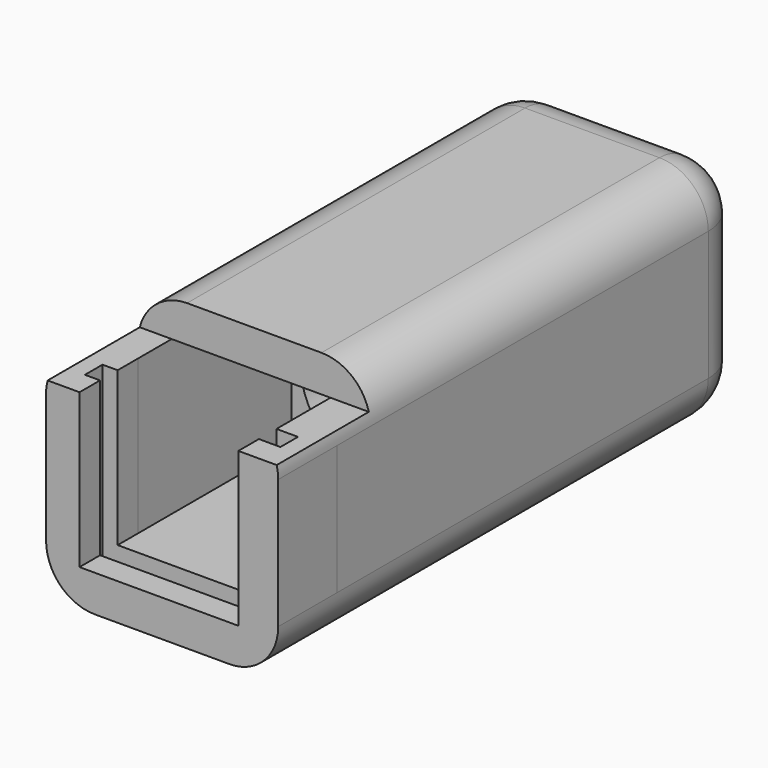
from build123d import *

# Parameters (mm, degrees)
F0_W         = 1.3692331631
F0_H         = 7.834737435
F0_W_2       = 6.5
F0_H_2       = 0.9
F0_W_3       = 0.6192331631
F0_H_3       = 1.05
F0_H_4       = 13.165262565
F0_W_4       = 0.8807668369
F0_W_5       = 1.6307668369
F1_DEPTH     = 0.9
F2_DEPTH     = 1.5
F3_DEPTH     = 7.8
F5_W         = 9.5
F5_H         = 19.2867757659
F6_DEPTH     = 1.5
F7_R         = 3
F8_DEPTH     = 20
F9_T1_DEPTH  = 5.3
F9_T3_DEPTH  = 5.5
F9_T5_DEPTH  = 22.2867757659
F9_T7_DEPTH  = 27
F9_S11_W     = 2
F9_S11_H     = 2
F9_T12_DEPTH = 2
F9_S17_W     = 2
F9_S17_H     = 2
F9_T18_DEPTH = 2
F9_S23_W     = 2
F9_S23_H     = 2
F9_T24_DEPTH = 2
F9_S29_W     = 2
F9_S29_H     = 2
F9_T30_DEPTH = 2
F10_R        = 2.7204865104
F11_DEPTH    = 6


# Not quite as in the source:
# - a fillet or chamfer that OpenCascade refuses, or shapes differently, is made with other operations: its cross-section is extruded or revolved along the edge and cut away or added
# - a feature names something its author has since deleted; it is built from what else it names


with BuildPart() as f1:
    # F0 (on Top) → F1 (new body)
    with BuildSketch(Plane.XY):
        Polygon((-4.75, 1.5), (-4.75, -1.5), (-3.3807668369, -1.5), (-3.3807668369, -0.45), (-4, -0.45), (-4, 0.45), (-3.3807668369, 0.45), (-3.3807668369, 1.5), align=None)
        Polygon((-3.3807668369, -0.45), (-3.3807668369, -1.5), (-3.1192331631, -1.5), (3.1192331631, -1.5), (3.1192331631, -0.45), align=None)
        with Locations((-4.0653834185, 5.4173687175)):
            Rectangle(F0_W, F0_H)
        with Locations((-0.1307668369, 0)):
            Rectangle(F0_W_2, F0_H_2)
        with Locations((-3.6903834185, 0)):
            Rectangle(F0_W_3, F0_H_2)
        with Locations((-0.1307668369, 5.4173687175)):
            Rectangle(F0_W_2, F0_H)
        with Locations((-0.1307668369, 0.975)):
            Rectangle(F0_W_2, F0_H_3)
        with Locations((-4.0653834185, 15.9173687175)):
            Rectangle(F0_W, F0_H_4)
        Polygon((3.1192331631, -0.45), (3.1192331631, -1.5), (3.3807668369, -1.5), (4.75, -1.5), (4.75, 1.5), (3.1192331631, 1.5), (3.1192331631, 0.45), (4, 0.45), (4, -0.45), align=None)
        with Locations((3.5596165815, 0)):
            Rectangle(F0_W_4, F0_H_2)
        with Locations((3.9346165815, 5.4173687175)):
            Rectangle(F0_W_5, F0_H)
        with Locations((-0.1307668369, 15.9173687175)):
            Rectangle(F0_W_2, F0_H_4)
        with Locations((3.9346165815, 15.9173687175)):
            Rectangle(F0_W_5, F0_H_4)
    extrude(amount=F1_DEPTH)

    # F0 (on Top) → F2 (join)
    with BuildSketch(Plane.XY):
        Polygon((-3.3807668369, -0.45), (-3.3807668369, -1.5), (-3.1192331631, -1.5), (3.1192331631, -1.5), (3.1192331631, -0.45), align=None)
        Polygon((3.1192331631, -0.45), (3.1192331631, -1.5), (3.3807668369, -1.5), (4.75, -1.5), (4.75, 1.5), (3.1192331631, 1.5), (3.1192331631, 0.45), (4, 0.45), (4, -0.45), align=None)
        Polygon((-4.75, 1.5), (-4.75, -1.5), (-3.3807668369, -1.5), (-3.3807668369, -0.45), (-4, -0.45), (-4, 0.45), (-3.3807668369, 0.45), (-3.3807668369, 1.5), align=None)
        with Locations((-0.1307668369, 0.975)):
            Rectangle(F0_W_2, F0_H_3)
        with Locations((-4.0653834185, 5.4173687175)):
            Rectangle(F0_W, F0_H)
        with Locations((3.9346165815, 5.4173687175)):
            Rectangle(F0_W_5, F0_H)
        with Locations((-0.1307668369, 5.4173687175)):
            Rectangle(F0_W_2, F0_H)
        with Locations((-4.0653834185, 15.9173687175)):
            Rectangle(F0_W, F0_H_4)
        with Locations((-0.1307668369, 15.9173687175)):
            Rectangle(F0_W_2, F0_H_4)
        with Locations((3.9346165815, 15.9173687175)):
            Rectangle(F0_W_5, F0_H_4)
    extrude(amount=F2_DEPTH)

    # F0 (on Top) → F3 (join)
    with BuildSketch(Plane.XY):
        Polygon((-4.75, 1.5), (-4.75, -1.5), (-3.3807668369, -1.5), (-3.3807668369, -0.45), (-4, -0.45), (-4, 0.45), (-3.3807668369, 0.45), (-3.3807668369, 1.5), align=None)
        Polygon((3.1192331631, -0.45), (3.1192331631, -1.5), (3.3807668369, -1.5), (4.75, -1.5), (4.75, 1.5), (3.1192331631, 1.5), (3.1192331631, 0.45), (4, 0.45), (4, -0.45), align=None)
        with Locations((-4.0653834185, 5.4173687175)):
            Rectangle(F0_W, F0_H)
        with Locations((3.9346165815, 5.4173687175)):
            Rectangle(F0_W_5, F0_H)
        with Locations((-4.0653834185, 15.9173687175)):
            Rectangle(F0_W, F0_H_4)
        with Locations((-0.1307668369, 15.9173687175)):
            Rectangle(F0_W_2, F0_H_4)
        with Locations((3.9346165815, 15.9173687175)):
            Rectangle(F0_W_5, F0_H_4)
    extrude(amount=F3_DEPTH)

    # F5 (on offset) → F6 (join)
    with BuildSketch(Plane.XY.offset(7.8)):
        with Locations((0, 12.856612117)):
            Rectangle(F5_W, F5_H)
    extrude(amount=F6_DEPTH)

    # F7 (on Front) → F8 (cut)
    with BuildSketch(Plane.XZ):
        with Locations((0, 4.5)):
            Circle(F7_R)
    extrude(amount=-F8_DEPTH, mode=Mode.SUBTRACT)

    # F9: fillet of radius 2 on 8 edges, made by hand

    # F9_s2 → F9_t1 (cut)
    with BuildSketch(Plane.XY.offset(2)):
        with BuildLine():
            ThreePointArc((4.75, 20.5), (4.1642135624, 21.9142135624), (2.75, 22.5))
            Line((2.75, 22.5), (4.75, 22.5))
            Line((4.75, 22.5), (4.75, 20.5))
        make_face()
        with BuildLine():
            ThreePointArc((-4.75, 20.5), (-4.1642135624, 21.9142135624), (-2.75, 22.5))
            Line((-2.75, 22.5), (-4.75, 22.5))
            Line((-4.75, 22.5), (-4.75, 20.5))
        make_face()
    extrude(amount=F9_T1_DEPTH, mode=Mode.SUBTRACT)

    # F9_s4 → F9_t3 (cut)
    with BuildSketch(Plane.YZ.offset(-2.75)):
        with BuildLine():
            ThreePointArc((20.5, 9.3), (21.9142135624, 8.7142135624), (22.5, 7.3))
            Line((22.5, 7.3), (22.5, 9.3))
            Line((22.5, 9.3), (20.5, 9.3))
        make_face()
        with BuildLine():
            ThreePointArc((20.5, 0), (21.9142135624, 0.5857864376), (22.5, 2))
            Line((22.5, 2), (22.5, 0))
            Line((22.5, 0), (20.5, 0))
        make_face()
    extrude(amount=F9_T3_DEPTH, mode=Mode.SUBTRACT)

    # F9_s6 → F9_t5 (cut)
    with BuildSketch(Plane.XZ.offset(-20.5)):
        with BuildLine():
            ThreePointArc((4.75, 7.3), (4.1642135624, 8.7142135624), (2.75, 9.3))
            Line((2.75, 9.3), (4.75, 9.3))
            Line((4.75, 9.3), (4.75, 7.3))
        make_face()
        with BuildLine():
            ThreePointArc((-4.75, 7.3), (-4.1642135624, 8.7142135624), (-2.75, 9.3))
            Line((-2.75, 9.3), (-4.75, 9.3))
            Line((-4.75, 9.3), (-4.75, 7.3))
        make_face()
    extrude(amount=F9_T5_DEPTH, mode=Mode.SUBTRACT)

    # F9_s8 → F9_t7 (cut)
    with BuildSketch(Plane.XZ.offset(-20.5)):
        with BuildLine():
            ThreePointArc((2.75, 0), (4.1642135624, 0.5857864376), (4.75, 2))
            Line((4.75, 2), (4.75, 0))
            Line((4.75, 0), (2.75, 0))
        make_face()
        with BuildLine():
            ThreePointArc((-4.75, 2), (-4.1642135624, 0.5857864376), (-2.75, 0))
            Line((-2.75, 0), (-4.75, 0))
            Line((-4.75, 0), (-4.75, 2))
        make_face()
    extrude(amount=F9_T7_DEPTH, mode=Mode.SUBTRACT)


with BuildPart() as f9_tool10:
    # F9_s11 → F9_t12 (new body)
    with BuildSketch(Plane.YZ.offset(2.75)):
        with Locations((21.5, 8.3)):
            Rectangle(F9_S11_W, F9_S11_H)
    extrude(amount=F9_T12_DEPTH)

    # F9_s13 → F9_t14 (revolve, cut)
    with BuildSketch(Plane(origin=(2.75, 20.5, 7.3), x_dir=(0, -0.7071067812, -0.7071067812), z_dir=(0, -0.7071067812, 0.7071067812))):
        with BuildLine():
            ThreePointArc((0, -2), (2, 0), (0, 2))
            Line((0, 2), (0, -2))
        make_face()
    revolve(axis=Axis((2.75, 20.5, 7.3), (1, 0, 0)), mode=Mode.SUBTRACT)


with BuildPart() as f1_1:
    add(f1.part)

    # F9_t9: cut F9_tool10
    add(f9_tool10.part, mode=Mode.SUBTRACT)


with BuildPart() as f9_tool16:
    # F9_s17 → F9_t18 (new body)
    with BuildSketch(Plane.XY.offset(2)):
        with Locations((3.75, 21.5)):
            Rectangle(F9_S17_W, F9_S17_H)
    extrude(amount=-F9_T18_DEPTH)

    # F9_s19 → F9_t20 (revolve, cut)
    with BuildSketch(Plane(origin=(2.75, 20.5, 2), x_dir=(-0.7071067812, -0.7071067812, 0), z_dir=(0.7071067812, -0.7071067812, 0))):
        with BuildLine():
            ThreePointArc((0, -2), (2, 0), (0, 2))
            Line((0, 2), (0, -2))
        make_face()
    revolve(axis=Axis((2.75, 20.5, 2), (0, 0, -1)), mode=Mode.SUBTRACT)


with BuildPart() as f1_2:
    add(f1_1.part)

    # F9_t15: cut F9_tool16
    add(f9_tool16.part, mode=Mode.SUBTRACT)


with BuildPart() as f9_tool22:
    # F9_s23 → F9_t24 (new body)
    with BuildSketch(Plane.YZ.offset(-2.75)):
        with Locations((21.5, 8.3)):
            Rectangle(F9_S23_W, F9_S23_H)
    extrude(amount=-F9_T24_DEPTH)

    # F9_s25 → F9_t26 (revolve, cut)
    with BuildSketch(Plane(origin=(-2.75, 20.5, 7.3), x_dir=(0, -0.7071067812, -0.7071067812), z_dir=(0, 0.7071067812, -0.7071067812))):
        with BuildLine():
            ThreePointArc((0, -2), (2, 0), (0, 2))
            Line((0, 2), (0, -2))
        make_face()
    revolve(axis=Axis((-2.75, 20.5, 7.3), (-1, 0, 0)), mode=Mode.SUBTRACT)


with BuildPart() as f1_3:
    add(f1_2.part)

    # F9_t21: cut F9_tool22
    add(f9_tool22.part, mode=Mode.SUBTRACT)


with BuildPart() as f9_tool28:
    # F9_s29 → F9_t30 (new body)
    with BuildSketch(Plane.YZ.offset(-2.75)):
        with Locations((21.5, 1)):
            Rectangle(F9_S29_W, F9_S29_H)
    extrude(amount=-F9_T30_DEPTH)

    # F9_s31 → F9_t32 (revolve, cut)
    with BuildSketch(Plane(origin=(-2.75, 20.5, 2), x_dir=(0, -0.7071067812, 0.7071067812), z_dir=(0, -0.7071067812, -0.7071067812))):
        with BuildLine():
            ThreePointArc((0, -2), (2, 0), (0, 2))
            Line((0, 2), (0, -2))
        make_face()
    revolve(axis=Axis((-2.75, 20.5, 2), (-1, 0, 0)), mode=Mode.SUBTRACT)


with BuildPart() as f1_4:
    add(f1_3.part)

    # F9_t27: cut F9_tool28
    add(f9_tool28.part, mode=Mode.SUBTRACT)

    # F10 (on Top) → F11 (cut)
    with BuildSketch(Plane.XY):
        with Locations((0, 17.4578037113)):
            Circle(F10_R)
    extrude(amount=F11_DEPTH, mode=Mode.SUBTRACT)


solid = f1_4.part
